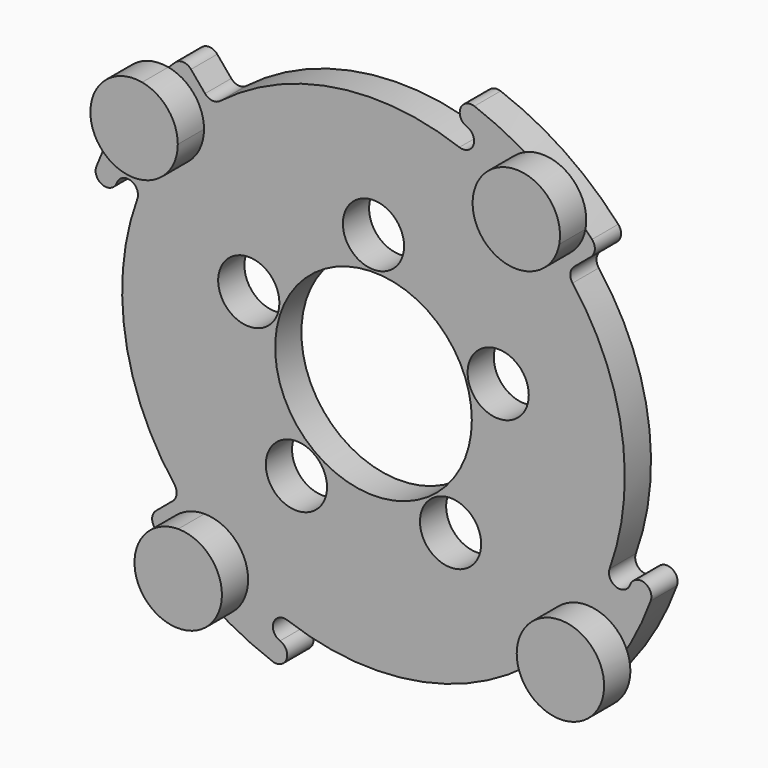
from build123d import *

# Parameters (mm, degrees)
F0_R     = 14
F0_R_2   = 45
F1_DEPTH = 15
F3_DEPTH = 15
F4_COUNT = 4


with BuildPart() as f1:
    # F0 (on Front) → F1 (new body)
    with BuildSketch(Plane.XZ):
        with BuildLine():
            ThreePointArc((-117.4615775982, 42.7525179157), (-111.0530137777, 45.740880303), (-108.0646513904, 39.3323164825))
            ThreePointArc((-108.0646513904, 39.3323164825), (-113.6444232454, -17.6052567496), (-91.0986302517, -70.1857504502))
            ThreePointArc((-91.0986302517, -70.1857504502), (-90.0886289945, -73.7767817278), (-91.8455022142, -77.0675270332))
            Line((-91.8455022142, -77.0675270332), (-99.5120922253, -83.500559884))
            ThreePointArc((-99.5120922253, -83.500559884), (-101.2865881138, -86.990889679), (-100.0019293376, -90.6896583342))
            ThreePointArc((-100.0019293376, -90.6896583342), (-75.2914558589, -112.0544362114), (-46.172719349, -126.8585038061))
            ThreePointArc((-46.172719349, -126.8585038061), (-39.7641555284, -123.8701414188), (-42.7525179157, -117.4615775982))
            ThreePointArc((-42.7525179157, -117.4615775982), (-45.740880303, -111.0530137777), (-39.3323164825, -108.0646513904))
            ThreePointArc((-39.3323164825, -108.0646513904), (17.6052567496, -113.6444232454), (70.1857504502, -91.0986302517))
            ThreePointArc((70.1857504502, -91.0986302517), (73.7767817278, -90.0886289945), (77.0675270332, -91.8455022142))
            Line((77.0675270332, -91.8455022142), (83.500559884, -99.5120922253))
            ThreePointArc((83.500559884, -99.5120922253), (86.990889679, -101.2865881138), (90.6896583342, -100.0019293376))
            ThreePointArc((90.6896583342, -100.0019293376), (112.0544362114, -75.2914558589), (126.8585038061, -46.172719349))
            ThreePointArc((126.8585038061, -46.172719349), (123.8701414188, -39.7641555284), (117.4615775982, -42.7525179157))
            ThreePointArc((117.4615775982, -42.7525179157), (111.0530137777, -45.740880303), (108.0646513904, -39.3323164825))
            ThreePointArc((108.0646513904, -39.3323164825), (113.6444232454, 17.6052567496), (91.0986302517, 70.1857504502))
            ThreePointArc((91.0986302517, 70.1857504502), (90.0886289945, 73.7767817278), (91.8455022142, 77.0675270332))
            Line((91.8455022142, 77.0675270332), (99.5120922253, 83.500559884))
            ThreePointArc((99.5120922253, 83.500559884), (101.2865881138, 86.990889679), (100.0019293376, 90.6896583342))
            ThreePointArc((100.0019293376, 90.6896583342), (75.2914558589, 112.0544362114), (46.172719349, 126.8585038061))
            ThreePointArc((46.172719349, 126.8585038061), (39.7641555284, 123.8701414188), (42.7525179157, 117.4615775982))
            ThreePointArc((42.7525179157, 117.4615775982), (45.740880303, 111.0530137777), (39.3323164825, 108.0646513904))
            ThreePointArc((39.3323164825, 108.0646513904), (-17.6052567496, 113.6444232454), (-70.1857504502, 91.0986302517))
            ThreePointArc((-70.1857504502, 91.0986302517), (-73.7767817278, 90.0886289945), (-77.0675270332, 91.8455022142))
            Line((-77.0675270332, 91.8455022142), (-83.500559884, 99.5120922253))
            ThreePointArc((-83.500559884, 99.5120922253), (-86.990889679, 101.2865881138), (-90.6896583342, 100.0019293376))
            ThreePointArc((-90.6896583342, 100.0019293376), (-112.0544362114, 75.2914558589), (-126.8585038061, 46.172719349))
            ThreePointArc((-126.8585038061, 46.172719349), (-123.8701414188, 39.7641555284), (-117.4615775982, 42.7525179157))
        make_face()
        with Locations((-35.2671151375, -48.5410196625)):
            Circle(F0_R, mode=Mode.SUBTRACT)
        with Locations((35.2671151375, -48.5410196625)):
            Circle(F0_R, mode=Mode.SUBTRACT)
        with Locations((-57.0633909777, 18.5410196625)):
            Circle(F0_R, mode=Mode.SUBTRACT)
        Circle(F0_R_2, mode=Mode.SUBTRACT)
        with Locations((57.0633909777, 18.5410196625)):
            Circle(F0_R, mode=Mode.SUBTRACT)
        with Locations((0, 60)):
            Circle(F0_R, mode=Mode.SUBTRACT)
    extrude(amount=F1_DEPTH)


with BuildPart() as f3:
    # F2 (on face) → F3 (new body)
    with BuildSketch(Plane.XZ.offset(15)):
        with BuildLine():
            ThreePointArc((-115.8535261196, 69.3033944743), (-105.7750972978, 83.8846159414), (-93.8731769133, 97.0197230269))
            ThreePointArc((-93.8731769133, 97.0197230269), (-113.2185300706, 89.7876074336), (-115.8535261196, 69.3033944743))
        make_face()
        with BuildLine():
            ThreePointArc((-115.8535261196, 69.3033944743), (-93.4315700512, 57.7884964424), (-77.5481452858, 77.3602569237))
            ThreePointArc((-77.5481452858, 77.3602569237), (-82.1614730099, 90.1372016397), (-93.8731769133, 97.0197230269))
            ThreePointArc((-93.8731769133, 97.0197230269), (-105.7750972978, 83.8846159414), (-115.8535261196, 69.3033944743))
        make_face()
    extrude(amount=F3_DEPTH)


with BuildPart() as f4_1:
    # F4: instance of F3
    add(f3.part.rotate(Axis((0, -15, 0), (0, -1, 0)), 1 * 360 / F4_COUNT))


with BuildPart() as f4_2:
    # F4: instance of F3
    add(f3.part.rotate(Axis((0, -15, 0), (0, -1, 0)), 2 * 360 / F4_COUNT))


with BuildPart() as f4_3:
    # F4: instance of F3
    add(f3.part.rotate(Axis((0, -15, 0), (0, -1, 0)), 3 * 360 / F4_COUNT))


solid = Compound([f1.part, f3.part, f4_1.part, f4_2.part, f4_3.part])
